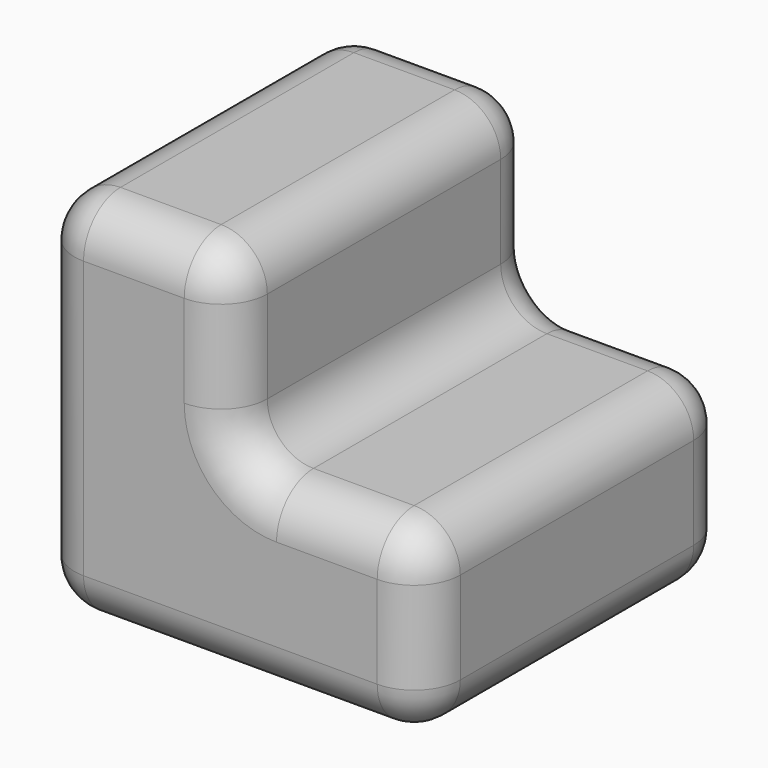
from build123d import *

# Parameters (mm, degrees)
F0_W     = 83.6216490716
F0_H     = 83.1985995173
F1_DEPTH = 40
F2_W     = 41.8108245358
F2_H     = 83.1985995173
F3_DEPTH = 40
F4_F1_R  = 10
F4_F2_R  = 10


with BuildPart() as f1:
    # F0 (on Top) → F1 (new body)
    with BuildSketch(Plane.XY):
        with Locations((-17.3164242879, -4.335001111)):
            Rectangle(F0_W, F0_H)
    extrude(amount=F1_DEPTH)

    # F2 (on face) → F3 (join)
    with BuildSketch(Plane.XY.offset(40)):
        with Locations((-38.2218365557, -4.335001111)):
            Rectangle(F2_W, F2_H)
    extrude(amount=F3_DEPTH)

    # F4: fillet of radius 10 on 16 edges, made by hand

    # F4_f1
    f4_f1_edges = [f1.edges().sort_by_distance(p)[0] for p in [
        (-17.3164242879, -4.335001111, 40),
    ]]
    fillet(f4_f1_edges, radius=F4_F1_R)

    # F4_f2
    f4_f2_edges = [f1.edges().sort_by_distance(p)[0] for p in [
        (-17.3164242879, -4.335001111, 80),
        (-38.2218365557, -45.9343008697, 80),
        (-17.3164242879, -45.9343008697, 65),
        (-59.1272488236, -4.335001111, 80),
        (-38.2218365557, 37.2642986476, 80),
        (8.58898798, 37.2642986476, 40),
        (24.4944002479, -4.335001111, 40),
        (24.4944002479, -45.9343008697, 20),
        (24.4944002479, 37.2642986476, 20),
        (-17.3164242879, -45.9343008697, 0),
        (-59.1272488236, -45.9343008697, 40),
        (-59.1272488236, 37.2642986476, 40),
        (-59.1272488236, -4.335001111, 0),
        (-17.3164242879, 37.2642986476, 0),
        (24.4944002479, -4.335001111, 0),
        (-14.3874920997, 37.2642986476, 42.9289321881),
        (-14.3874920997, -45.9343008697, 42.9289321881),
    ]]
    fillet(f4_f2_edges, radius=F4_F2_R)


solid = f1.part
